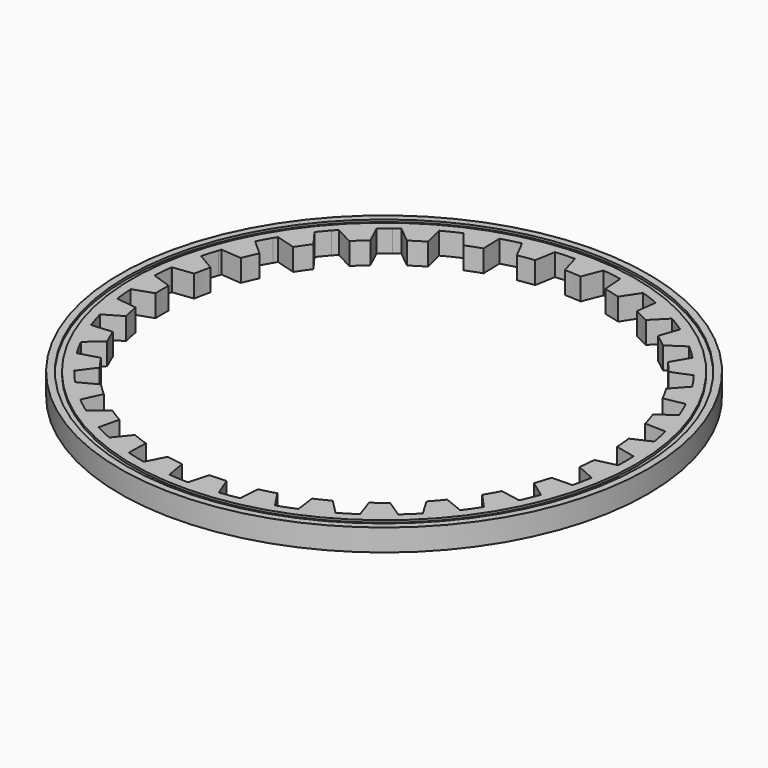
from build123d import *

# Parameters (mm, degrees)
F0_R            = 304.8
F1_DEPTH        = 25.4
F2_DEPTH        = 25.4
F2_COPIES_COUNT = 31
F3_R            = 296.8625
F3_R_2          = 290.5125
F4_DEPTH        = 2.54
F5_R            = 296.8625
F5_R_2          = 290.5125
F6_DEPTH        = 2.54


# Not quite as in the source:
# - a pattern or mirror of a feature is missing from the dataset's text; its kind, count and spacing are read off the source's solid


with BuildPart() as f1:
    # F0 (on Top) → F1 (new body)
    with BuildSketch(Plane.XY):
        Circle(F0_R)
        with BuildLine():
            ThreePointArc((-139.9074929569, 241.8475830239), (139.5962149699, 242.0273884627), (279.4, 0))
            ThreePointArc((279.4, 0), (8.5793400064, -279.2682490457), (-278.873120437, -17.1505888444))
            Line((-278.873120437, -17.1505888444), (-284.48, -19.05))
            Line((-284.48, -19.05), (-284.48, 19.05))
            Line((-284.48, 19.05), (-278.873120437, 17.1505888444))
            ThreePointArc((-278.873120437, 17.1505888444), (-278.0539903617, 27.392306291), (-276.8588574341, 37.5969820635))
            Line((-276.8588574341, 37.5969820635), (-282.7052908844, 36.7727961626))
            Line((-282.7052908844, 36.7727961626), (-275.2642057328, 74.52500298))
            Line((-275.2642057328, 74.52500298), (-270.0959710932, 71.5019328355))
            ThreePointArc((-270.0959710932, 71.5019328355), (-267.303871456, 81.3203560288), (-264.1549850662, 91.0302359916))
            Line((-264.1549850662, 91.0302359916), (-270.1311147854, 91.3975495928))
            Line((-270.1311147854, 91.3975495928), (-255.2871620754, 126.8976403584))
            Line((-255.2871620754, 126.8976403584), (-250.8902083052, 122.9571607373))
            ThreePointArc((-250.8902083052, 122.9571607373), (-246.2317976323, 132.0388648646), (-241.2447866782, 140.9443610102))
            Line((-241.2447866782, 140.9443610102), (-247.0326592074, 142.4729997596))
            Line((-247.0326592074, 142.4729997596), (-225.5328396666, 174.384889715))
            Line((-225.5328396666, 174.384889715), (-221.9907783353, 169.6598194449))
            ThreePointArc((-221.9907783353, 169.6598194449), (-215.6401479473, 177.6617195494), (-209.0012374477, 185.4261112825))
            Line((-209.0012374477, 185.4261112825), (-214.453995901, 188.1291797331))
            Line((-214.453995901, 188.1291797331), (-187.0092810122, 215.058314286))
            Line((-187.0092810122, 215.058314286), (-184.5245635336, 209.7976297595))
            ThreePointArc((-184.5245635336, 209.7976297595), (-176.734130204, 216.4010333179), (-168.7075759898, 222.715320092))
            Line((-168.7075759898, 222.715320092), (-173.4326522734, 226.2997079893))
            Line((-173.4326522734, 226.2997079893), (-141.3964217588, 247.6183643131))
            Line((-141.3964217588, 247.6183643131), (-139.9074929569, 241.8475830239))
        make_face(mode=Mode.SUBTRACT)
        with BuildLine():
            ThreePointArc((-241.2447866782, 140.9443610102), (-232.0623656728, 155.6001877838), (-221.9907783353, 169.6598194449))
            Line((-221.9907783353, 169.6598194449), (-225.5328396666, 174.384889715))
            Line((-225.5328396666, 174.384889715), (-247.0326592074, 142.4729997596))
            Line((-247.0326592074, 142.4729997596), (-241.2447866782, 140.9443610102))
        make_face()
        with BuildLine():
            ThreePointArc((-209.0012374477, 185.4261112825), (-197.1398786083, 197.9904751807), (-184.5245635336, 209.7976297595))
            Line((-184.5245635336, 209.7976297595), (-187.0092810122, 215.058314286))
            Line((-187.0092810122, 215.058314286), (-214.453995901, 188.1291797331))
            Line((-214.453995901, 188.1291797331), (-209.0012374477, 185.4261112825))
        make_face()
        with BuildLine():
            ThreePointArc((-168.7075759898, 222.715320092), (-154.603771191, 232.7273811427), (-139.9074929569, 241.8475830239))
            Line((-139.9074929569, 241.8475830239), (-141.3964217588, 247.6183643131))
            Line((-141.3964217588, 247.6183643131), (-173.4326522734, 226.2997079893))
            Line((-173.4326522734, 226.2997079893), (-168.7075759898, 222.715320092))
        make_face()
        with BuildLine():
            Line((-270.1311147854, 91.3975495928), (-264.1549850662, 91.0302359916))
            ThreePointArc((-264.1549850662, 91.0302359916), (-258.0168985448, 107.1990674648), (-250.8902083052, 122.9571607373))
            Line((-250.8902083052, 122.9571607373), (-255.2871620754, 126.8976403584))
            Line((-255.2871620754, 126.8976403584), (-270.1311147854, 91.3975495928))
        make_face()
        with BuildLine():
            Line((-282.7052908844, 36.7727961626), (-276.8588574341, 37.5969820635))
            ThreePointArc((-276.8588574341, 37.5969820635), (-274.0023403806, 54.6541623845), (-270.0959710932, 71.5019328355))
            Line((-270.0959710932, 71.5019328355), (-275.2642057328, 74.52500298))
            Line((-275.2642057328, 74.52500298), (-282.7052908844, 36.7727961626))
        make_face()
        with BuildLine():
            Line((-284.48, -19.05), (-278.873120437, -17.1505888444))
            ThreePointArc((-278.873120437, -17.1505888444), (-279.4, 0), (-278.873120437, 17.1505888444))
            Line((-278.873120437, 17.1505888444), (-284.48, 19.05))
            Line((-284.48, 19.05), (-284.48, -19.05))
        make_face()
    extrude(amount=F1_DEPTH)

    # F0 (on Top) → F2 (join)
    with BuildSketch(Plane.XY):
        with BuildLine():
            ThreePointArc((-278.873120437, 17.1505888444), (-279.4, 0), (-278.873120437, -17.1505888444))
            Line((-278.873120437, -17.1505888444), (-256.3631135226, -9.525))
            ThreePointArc((-256.3631135226, -9.525), (-256.54, 0), (-256.3631135226, 9.525))
            Line((-256.3631135226, 9.525), (-278.873120437, 17.1505888444))
        make_face()
    f2 = extrude(amount=F2_DEPTH)

    # F2_copies: F2 ×31 about axis
    f2_copies_axis = Axis((0, 0, 0), (0, 0, 1))
    for i in range(1, F2_COPIES_COUNT):
        add(f2.rotate(f2_copies_axis, i * 360 / F2_COPIES_COUNT))

    # F3 (on face) → F4 (cut)
    with BuildSketch(Plane(origin=(0, 0, 0), x_dir=(1, 0, 0), z_dir=(0, 0, -1))):
        Circle(F3_R)
        Circle(F3_R_2, mode=Mode.SUBTRACT)
    extrude(amount=-F4_DEPTH, mode=Mode.SUBTRACT)

    # F5 (on face) → F6 (cut)
    with BuildSketch(Plane.XY.offset(25.4)):
        Circle(F5_R)
        Circle(F5_R_2, mode=Mode.SUBTRACT)
    extrude(amount=-F6_DEPTH, mode=Mode.SUBTRACT)


solid = f1.part
